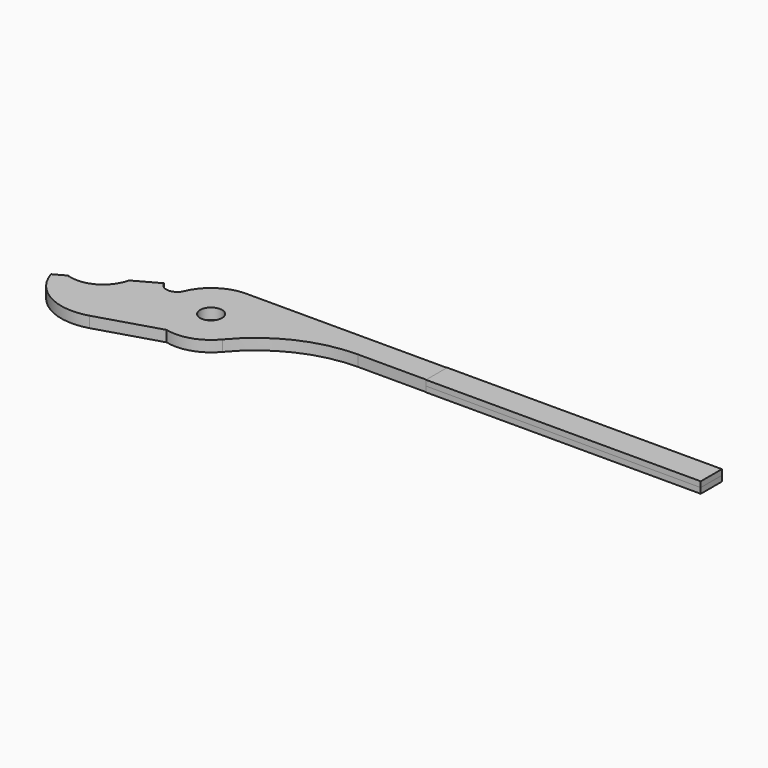
from build123d import *

# Parameters (mm, degrees)
F1_R     = 3.1736948077
F2_DEPTH = 1.5875
F3_DEPTH = 1.5875
F4_DEPTH = 1.5875
F6_DEPTH = 25.4


with BuildPart() as f2:
    # F1 (on face) → F2 (new body)
    with BuildSketch(Plane.XY):
        with BuildLine():
            ThreePointArc((-40.3451274018, -7.3844323762), (-32.7517807814, -16.6165715435), (-20.8546804416, -17.7785999452))
            Line((-20.8546804416, -17.7785999452), (-2.9840807938, -12.3444425478))
            ThreePointArc((-2.9840807938, -12.3444425478), (3.9996215585, -12.0537557379), (9.771792507, -8.1118475823))
            ThreePointArc((9.771792507, -8.1118475823), (22.5181286005, 1.749315086), (38.2470712066, 5.2581578403))
            Line((38.2470712066, 5.2581578403), (57.9611142654, 5.2581578403))
            Line((57.9611142654, 5.2581578403), (57.9611142654, 12.7))
            Line((57.9611142654, 12.7), (0, 12.7))
            ThreePointArc((0, 12.7), (-7.0383356023, 10.5712739038), (-11.7171926739, 4.8987136927))
            ThreePointArc((-11.7171926739, 4.8987136927), (-14.7583668014, 2.950363788), (-17.6547681255, 5.1080632099))
            Line((-17.6547681255, 5.1080632099), (-24.7176810189, 1.2194774422))
            ThreePointArc((-24.7176810189, 1.2194774422), (-29.3095141905, -4.8881094223), (-36.925990654, -5.5019786781))
            Line((-36.925990654, -5.5019786781), (-40.3451274018, -7.3844323762))
        make_face()
        Circle(F1_R, mode=Mode.SUBTRACT)
    extrude(amount=F2_DEPTH)

    # F3 (add): a face of the model
    f3_faces = [f2.faces().sort_by_distance(p)[0] for p in [
        (-6.4668185994, 9.7128802267, 1.5875),
    ]]
    extrude(f3_faces, amount=F3_DEPTH)

    # F5 (on face) → F6 (cut)
    with BuildSketch(Plane.XY.offset(3.175)):
        with BuildLine():
            ThreePointArc((-36.2762714732, -5.7071182517), (-36.4439228923, -5.6591640871), (-36.6106467962, -5.6080784715))
            Line((-36.6106467962, -5.6080784715), (-36.6106467962, -5.954187482))
            Line((-36.6106467962, -5.954187482), (-36.2762714732, -5.7071182517))
        make_face()
    extrude(amount=-F6_DEPTH, mode=Mode.SUBTRACT)


with BuildPart() as f2b:
    # F0 (on Top) → F2, piece 2 (new body)
    with BuildSketch(Plane.XY):
        Polygon((57.9611142654, 12.7), (57.9611142654, 5.2581578403), (57.9611142654, 5.1571133081), (137.3361142654, 5.1571133081), (137.3361142654, 12.8025133081), (57.9611142654, 12.8025133081), align=None)
    extrude(amount=F2_DEPTH)


with BuildPart() as f4:
    # F4 (new): a face of the model
    f4_faces = [f2b.part.faces().sort_by_distance(p)[0] for p in [
        (97.6486142654, 8.9798133081, 1.5875),
    ]]
    extrude(f4_faces, amount=F4_DEPTH)


solid = Compound([f2.part, f2b.part, f4.part])
